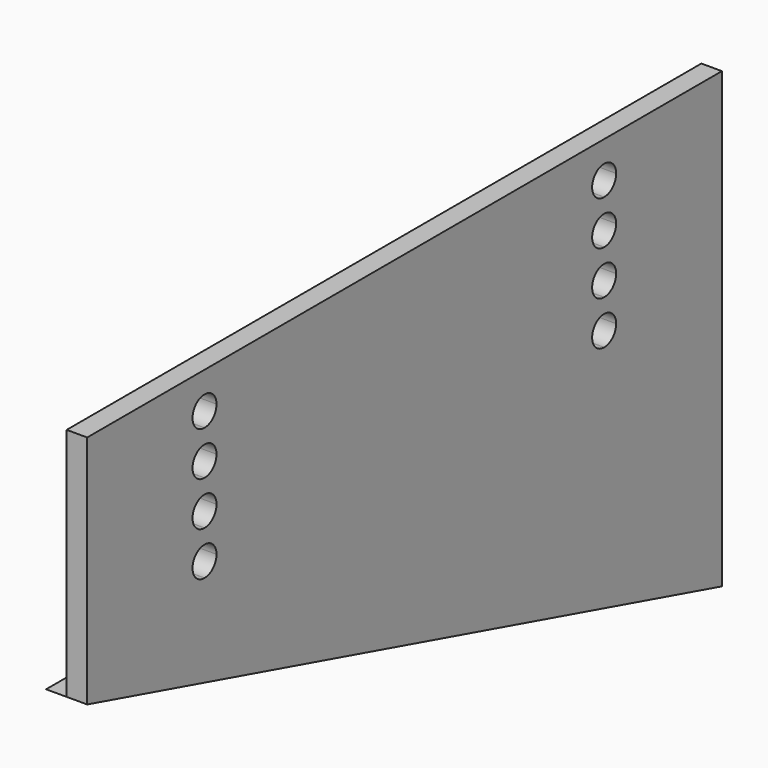
from build123d import *

# Parameters (mm, degrees)
F1_DEPTH = 7
F3_DEPTH = 7


# Not quite as in the source:
# - a feature names something its author has since deleted; it is built from what else it names


with BuildPart() as f1:
    # F0 (on Right) → F1 (new body)
    with BuildSketch(Plane.YZ):
        Polygon((-102.4108821703, 80), (-152.4108821703, 80), (-152.4108821703, 0), (117.5891178297, 0), (117.5891178297, 80), (67.5891178297, 80), align=None)
        with BuildLine():
            ThreePointArc((-102.4608821703, 27.6177177185), (-98.8930703505, 26.1711353257), (-97.4108821703, 22.6179677248))
            ThreePointArc((-97.4108821703, 22.6179677248), (-98.8930703505, 19.0648001239), (-102.4608821703, 17.6182177311))
            ThreePointArc((-102.4608821703, 17.6182177311), (-102.5108821703, 17.6179677248), (-102.5608821703, 17.6182177311))
            ThreePointArc((-102.5608821703, 17.6182177311), (-107.6108821703, 22.6179677248), (-102.5608821703, 27.6177177185))
            ThreePointArc((-102.5608821703, 27.6177177185), (-102.5108821703, 27.6179677248), (-102.4608821703, 27.6177177185))
        make_face(mode=Mode.SUBTRACT)
        with BuildLine():
            ThreePointArc((-102.4608821703, 42.6177177185), (-98.8930703505, 41.1711353257), (-97.4108821703, 37.6179677248))
            ThreePointArc((-97.4108821703, 37.6179677248), (-98.8930703505, 34.0648001239), (-102.4608821703, 32.6182177311))
            ThreePointArc((-102.4608821703, 32.6182177311), (-102.5108821703, 32.6179677248), (-102.5608821703, 32.6182177311))
            ThreePointArc((-102.5608821703, 32.6182177311), (-107.6108821703, 37.6179677248), (-102.5608821703, 42.6177177185))
            ThreePointArc((-102.5608821703, 42.6177177185), (-102.5108821703, 42.6179677248), (-102.4608821703, 42.6177177185))
        make_face(mode=Mode.SUBTRACT)
        with BuildLine():
            ThreePointArc((-102.4608821703, 57.6177177185), (-98.8930703505, 56.1711353257), (-97.4108821703, 52.6179677248))
            ThreePointArc((-97.4108821703, 52.6179677248), (-98.8930703505, 49.0648001239), (-102.4608821703, 47.6182177311))
            ThreePointArc((-102.4608821703, 47.6182177311), (-102.5108821703, 47.6179677248), (-102.5608821703, 47.6182177311))
            ThreePointArc((-102.5608821703, 47.6182177311), (-107.6108821703, 52.6179677248), (-102.5608821703, 57.6177177185))
            ThreePointArc((-102.5608821703, 57.6177177185), (-102.5108821703, 57.6179677248), (-102.4608821703, 57.6177177185))
        make_face(mode=Mode.SUBTRACT)
        with BuildLine():
            ThreePointArc((-102.4608821703, 72.6177177185), (-98.8930703505, 71.1711353257), (-97.4108821703, 67.6179677248))
            ThreePointArc((-97.4108821703, 67.6179677248), (-98.8930703505, 64.0648001239), (-102.4608821703, 62.6182177311))
            ThreePointArc((-102.4608821703, 62.6182177311), (-102.5108821703, 62.6179677248), (-102.5608821703, 62.6182177311))
            ThreePointArc((-102.5608821703, 62.6182177311), (-107.6108821703, 67.6179677248), (-102.5608821703, 72.6177177185))
            ThreePointArc((-102.5608821703, 72.6177177185), (-102.5108821703, 72.6179677248), (-102.4608821703, 72.6177177185))
        make_face(mode=Mode.SUBTRACT)
        with BuildLine():
            ThreePointArc((67.5391178297, 27.6177177185), (71.1069296495, 26.1711353257), (72.5891178297, 22.6179677248))
            ThreePointArc((72.5891178297, 22.6179677248), (71.1069296495, 19.0648001239), (67.5391178297, 17.6182177311))
            ThreePointArc((67.5391178297, 17.6182177311), (67.4891178297, 17.6179677248), (67.4391178297, 17.6182177311))
            ThreePointArc((67.4391178297, 17.6182177311), (62.3891178297, 22.6179677248), (67.4391178297, 27.6177177185))
            ThreePointArc((67.4391178297, 27.6177177185), (67.4891178297, 27.6179677248), (67.5391178297, 27.6177177185))
        make_face(mode=Mode.SUBTRACT)
        with BuildLine():
            ThreePointArc((67.5391178297, 42.6177177185), (71.1069296495, 41.1711353257), (72.5891178297, 37.6179677248))
            ThreePointArc((72.5891178297, 37.6179677248), (71.1069296495, 34.0648001239), (67.5391178297, 32.6182177311))
            ThreePointArc((67.5391178297, 32.6182177311), (67.4891178297, 32.6179677248), (67.4391178297, 32.6182177311))
            ThreePointArc((67.4391178297, 32.6182177311), (62.3891178297, 37.6179677248), (67.4391178297, 42.6177177185))
            ThreePointArc((67.4391178297, 42.6177177185), (67.4891178297, 42.6179677248), (67.5391178297, 42.6177177185))
        make_face(mode=Mode.SUBTRACT)
        with BuildLine():
            ThreePointArc((67.5391178297, 57.6177177185), (71.1069296495, 56.1711353257), (72.5891178297, 52.6179677248))
            ThreePointArc((72.5891178297, 52.6179677248), (71.1069296495, 49.0648001239), (67.5391178297, 47.6182177311))
            ThreePointArc((67.5391178297, 47.6182177311), (67.4891178297, 47.6179677248), (67.4391178297, 47.6182177311))
            ThreePointArc((67.4391178297, 47.6182177311), (62.3891178297, 52.6179677248), (67.4391178297, 57.6177177185))
            ThreePointArc((67.4391178297, 57.6177177185), (67.4891178297, 57.6179677248), (67.5391178297, 57.6177177185))
        make_face(mode=Mode.SUBTRACT)
        with BuildLine():
            ThreePointArc((67.5391178297, 72.6177177185), (71.1069296495, 71.1711353257), (72.5891178297, 67.6179677248))
            ThreePointArc((72.5891178297, 67.6179677248), (71.1069296495, 64.0648001239), (67.5391178297, 62.6182177311))
            ThreePointArc((67.5391178297, 62.6182177311), (67.4891178297, 62.6179677248), (67.4391178297, 62.6182177311))
            ThreePointArc((67.4391178297, 62.6182177311), (62.3891178297, 67.6179677248), (67.4391178297, 72.6177177185))
            ThreePointArc((67.4391178297, 72.6177177185), (67.4891178297, 72.6179677248), (67.5391178297, 72.6177177185))
        make_face(mode=Mode.SUBTRACT)
        Polygon((117.5891178297, 0), (-152.4108821703, 0), (117.5891178297, -74.3703905304), align=None)
    extrude(amount=F1_DEPTH)

    # F2 (on face) → F3 (join)
    with BuildSketch(Plane(origin=(0, 0, 0), x_dir=(0, -1, 0), z_dir=(-1, 0, 0))):
        Polygon((-117.5891178297, -74.3703905304), (152.4108821703, 0), (-117.5891178297, 0), align=None)
    extrude(amount=F3_DEPTH)


solid = f1.part
